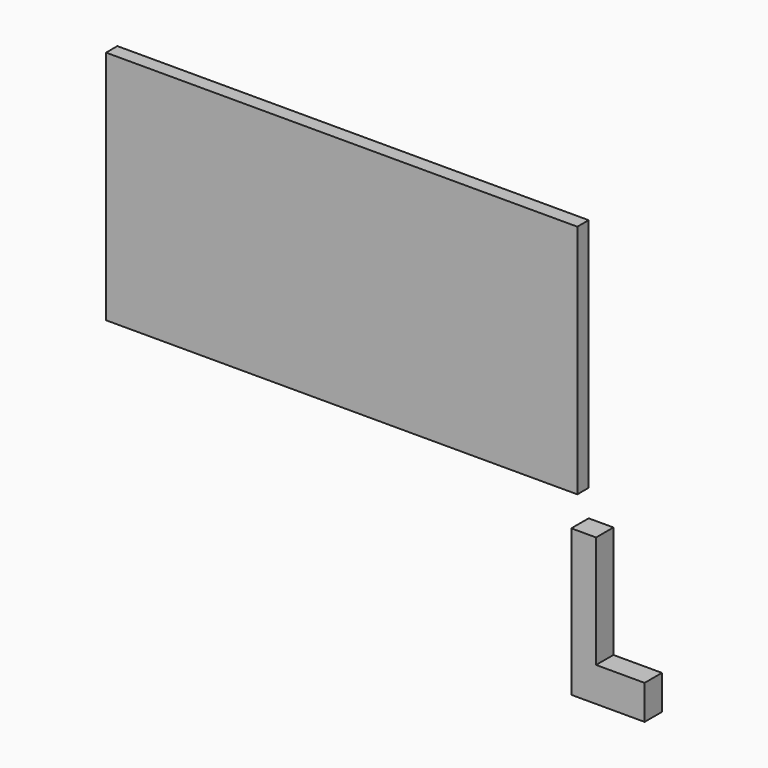
from build123d import *

# Parameters (mm, degrees)
F0_W     = 100
F0_H     = 50
F1_DEPTH = 3
F3_DEPTH = 4.6


# Not quite as in the source:
# - a feature names something its author has since deleted; it is built from what else it names


with BuildPart() as f1:
    # F0 (on Front) → F1 (new body)
    with BuildSketch(Plane.XZ):
        with Locations((-50, 25)):
            Rectangle(F0_W, F0_H)
    extrude(amount=F1_DEPTH)


with BuildPart() as f3:
    # F2 (on Front) → F3 (new body)
    with BuildSketch(Plane.XZ):
        Polygon((5.2557173185, -5.6901420467), (0, -5.6901420467), (0, -36.7995537817), (15.5540080741, -36.7995537817), (15.5540080741, -29.5049361885), (5.2557173185, -29.5049361885), align=None)
    extrude(amount=F3_DEPTH)


solid = Compound([f1.part, f3.part])
